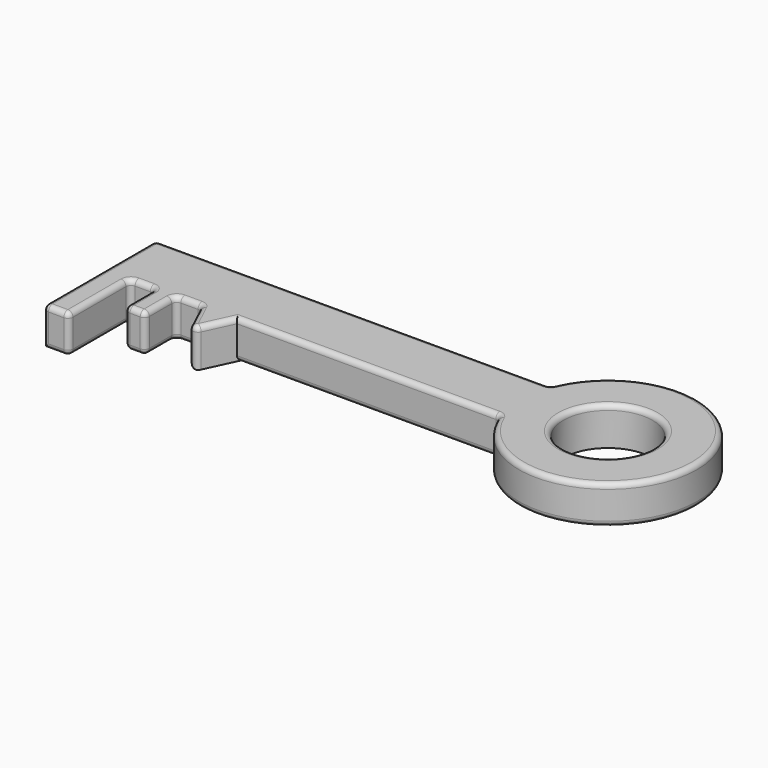
from build123d import *

# Parameters (mm, degrees)
F0_W     = 10
F0_H     = 30
F0_W_2   = 8
F0_H_2   = 15
F0_R     = 17.5
F1_DEPTH = 15
F2_F1_R  = 2
F2_F2_R  = 2


with BuildPart() as f1:
    # F0 (on Top) → F1 (new body)
    with BuildSketch(Plane.XY):
        Polygon((0, 9.9814090133), (-155, 9.9814090133), (-155, -15.0185909867), (-145, -15.0185909867), (-135, -15.0185909867), (-127, -15.0185909867), (-117, -15.0185909867), (-103, -15.0185909867), (0, -15.0185909867), align=None)
        with Locations((-150, -30.0185909867)):
            Rectangle(F0_W, F0_H)
        with Locations((-131, -22.5185909867)):
            Rectangle(F0_W_2, F0_H_2)
        Polygon((-110, -30.0185909867), (-103, -15.0185909867), (-117, -15.0185909867), align=None)
        with BuildLine():
            ThreePointArc((0, -15.0185909867), (67.6917420766, -2.5185909867), (0, 9.9814090133))
            Line((0, 9.9814090133), (0, -15.0185909867))
        make_face()
        with Locations((32.6917420766, -2.5185909867)):
            Circle(F0_R, mode=Mode.SUBTRACT)
    extrude(amount=F1_DEPTH)

    # F2: fillet of radius 2 on 33 edges, made by hand

    # F2_f1
    f2_f1_edges = [f1.edges().sort_by_distance(p)[0] for p in [
        (-117, -15.0185909867, 7.5),
        (-145, -15.0185909867, 7.5),
        (-135, -15.0185909867, 7.5),
        (-127, -15.0185909867, 7.5),
        (0, -15.0185909867, 7.5),
        (0, 9.9814090133, 7.5),
    ]]
    fillet(f2_f1_edges, radius=F2_F1_R)

    # F2_f2
    f2_f2_edges = [f1.edges().sort_by_distance(p)[0] for p in [
        (-78.1743375386, 9.9814090133, 15),
        (-155, -17.5185909867, 15),
        (-145, -31.0185909867, 15),
        (-140, -15.0185909867, 15),
        (-135, -23.5185909867, 15),
        (-127, -23.5185909867, 15),
        (-131, -30.0185909867, 15),
        (-113.2306798838, -23.0957055214, 15),
        (-52.1743375386, -15.0185909867, 15),
        (-106.5, -22.5185909867, 15),
        (67.6917420766, -2.5185909867, 15),
        (15.1917420766, -2.5185909867, 15),
        (-135, -30.0185909867, 7.5),
        (-127, -30.0185909867, 7.5),
        (-131, -30.0185909867, 0),
        (-140, -15.0185909867, 0),
        (-155, -45.0185909867, 7.5),
        (-145, -45.0185909867, 7.5),
        (-150, -45.0185909867, 0),
        (-150, -45.0185909867, 15),
        (-121.6368630238, -15.0185909867, 0),
        (-121.6368630238, -15.0185909867, 15),
        (-110, -30.0185909867, 7.5),
        (-113.2306798838, -23.0957055214, 0),
        (67.6917420766, -2.5185909867, 0),
        (-155, 9.9814090133, 7.5),
        (-78.1743375386, 9.9814090133, 0),
        (-0.245853144, 10.3129415177, 0),
        (-0.245853144, -15.3501234912, 0),
        (-117.1993755139, -15.3316496924, 0),
        (-126.4142135624, -15.6043774244, 15),
        (-117.1993755139, -15.3316496924, 15),
        (-126.4142135624, -15.6043774244, 0),
        (-144.4142135624, -15.6043774244, 0),
        (-135.5857864376, -15.6043774244, 0),
        (-0.245853144, -15.3501234912, 15),
        (-0.245853144, 10.3129415177, 15),
        (-135.5857864376, -15.6043774244, 15),
        (-144.4142135624, -15.6043774244, 15),
    ]]
    fillet(f2_f2_edges, radius=F2_F2_R)


solid = f1.part
